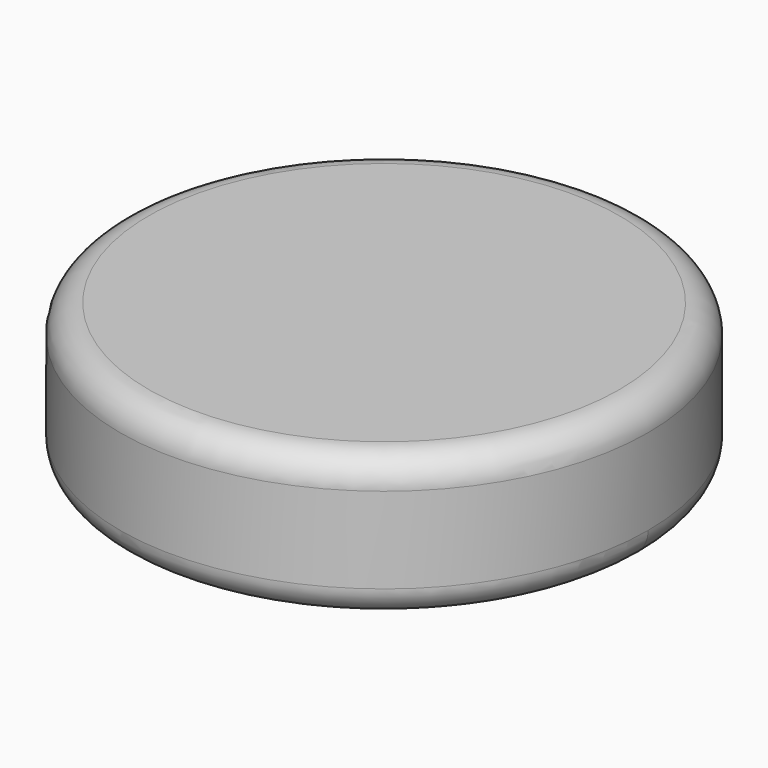
from build123d import *

# Parameters (mm, degrees)
F0_R         = 46.814869955
F1_DEPTH     = 25.4
F2_R         = 5.08
F3_TEXT_SIZE = 70.5555555556
F4_DEPTH     = 12.7


# Not quite as in the source:
# - Text() gives the source's letters only with a copy of the font that has no kerning and outlines rounded to 1/6400 em; it was checked with that copy


with BuildPart() as f1:
    # F0 (on Top) → F1 (new body)
    with BuildSketch(Plane.XY):
        Circle(F0_R)
    extrude(amount=F1_DEPTH)

    # F2
    f2_edges = [f1.edges().sort_by_distance(p)[0] for p in [
        (-46.81487, 0, 0),
        (-46.81487, 0, 25.4),
    ]]
    fillet(f2_edges, radius=F2_R)

    # F3 (on Top) → F4 (cut)
    with BuildSketch(Plane.XY):
        with Locations((-18.1579834821, -2.2900940815)):
            Text('1', F3_TEXT_SIZE, font='Open Sans', text_align=(TextAlign.LEFT, TextAlign.BOTTOM))
    extrude(amount=F4_DEPTH, mode=Mode.SUBTRACT)


solid = f1.part
